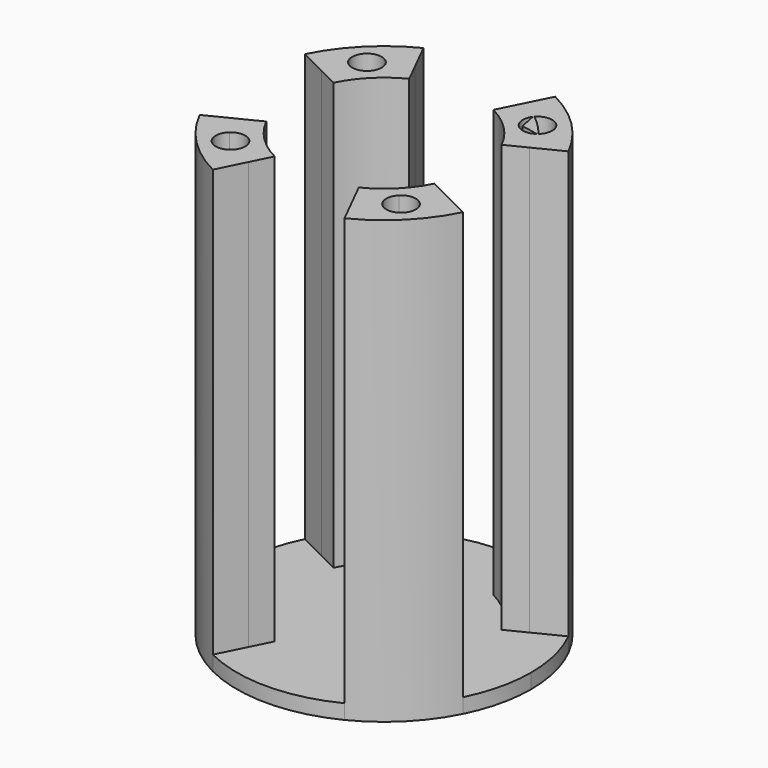
from build123d import *
from build123d import SkipClean  # not in build123d's __all__

# Parameters (mm, degrees)
F1_DEPTH = 5.08
F2_DEPTH = 152.4
F4_DEPTH = 50.8


with BuildPart() as f1:
    # F0 (on Top) → F1 (new body)
    with BuildSketch(Plane.XY):
        with BuildLine():
            Line((-29.00712, 14.50356), (0, 0))
            Line((0, 0), (-14.50356, 29.00712))
            ThreePointArc((-14.50356, 29.00712), (-22.932142, 22.932142), (-29.00712, 14.50356))
        make_face()
        with BuildLine():
            Line((-14.50356, 29.00712), (0, 0))
            Line((0, 0), (0, 32.430946))
            ThreePointArc((0, 32.430946), (-7.451105, 31.563386), (-14.50356, 29.00712))
        make_face()
        with BuildLine():
            Line((0, 32.430946), (0, 0))
            Line((0, 0), (14.50356, 29.00712))
            ThreePointArc((14.50356, 29.00712), (7.451105, 31.563386), (0, 32.430946))
        make_face()
        with BuildLine():
            Line((14.50356, 29.00712), (0, 0))
            Line((0, 0), (22.932142, 22.932142))
            ThreePointArc((22.932142, 22.932142), (18.962708, 26.309352), (14.50356, 29.00712))
        make_face()
        with BuildLine():
            Line((22.932142, 22.932142), (0, 0))
            Line((0, 0), (29.00712, 14.50356))
            ThreePointArc((29.00712, 14.50356), (26.309352, 18.962708), (22.932142, 22.932142))
        make_face()
        with BuildLine():
            Line((29.00712, 14.50356), (0, 0))
            Line((0, 0), (32.430946, 0))
            ThreePointArc((32.430946, 0), (31.563386, 7.451105), (29.00712, 14.50356))
        make_face()
        with BuildLine():
            Line((32.430946, 0), (0, 0))
            Line((0, 0), (29.00712, -14.50356))
            ThreePointArc((29.00712, -14.50356), (31.563386, -7.451105), (32.430946, 0))
        make_face()
        with BuildLine():
            Line((29.00712, -14.50356), (0, 0))
            Line((0, 0), (14.50356, -29.00712))
            ThreePointArc((14.50356, -29.00712), (22.932142, -22.932142), (29.00712, -14.50356))
        make_face()
        with BuildLine():
            Line((14.50356, -29.00712), (0, 0))
            Line((0, 0), (-14.50356, -29.00712))
            ThreePointArc((-14.50356, -29.00712), (0, -32.430946), (14.50356, -29.00712))
        make_face()
        with BuildLine():
            Line((-14.50356, -29.00712), (0, 0))
            Line((0, 0), (-29.00712, -14.50356))
            ThreePointArc((-29.00712, -14.50356), (-22.932142, -22.932142), (-14.50356, -29.00712))
        make_face()
        with BuildLine():
            Line((-29.00712, -14.50356), (0, 0))
            Line((0, 0), (-29.00712, 14.50356))
            ThreePointArc((-29.00712, 14.50356), (-32.430946, 0), (-29.00712, -14.50356))
        make_face()
        with BuildLine():
            ThreePointArc((-29.00712, -14.50356), (-32.430946, 0), (-29.00712, 14.50356))
            Line((-29.00712, 14.50356), (-35.921024, 17.960512))
            ThreePointArc((-35.921024, 17.960512), (-40.160926, 0), (-35.921024, -17.960512))
            Line((-35.921024, -17.960512), (-29.00712, -14.50356))
        make_face()
        with BuildLine():
            ThreePointArc((-29.00712, 14.50356), (-22.932142, 22.932142), (-14.50356, 29.00712))
            Line((-14.50356, 29.00712), (-17.960512, 35.921024))
            ThreePointArc((-17.960512, 35.921024), (-28.398063, 28.398063), (-35.921024, 17.960512))
            Line((-35.921024, 17.960512), (-29.00712, 14.50356))
        make_face()
        with BuildLine():
            ThreePointArc((-14.50356, 29.00712), (-7.451105, 31.563386), (0, 32.430946))
            Line((0, 32.430946), (0, 35.921024))
            Line((0, 35.921024), (17.960512, 35.921024))
            ThreePointArc((17.960512, 35.921024), (0, 40.160926), (-17.960512, 35.921024))
            Line((-17.960512, 35.921024), (-14.50356, 29.00712))
        make_face()
        with BuildLine():
            Line((0, 35.921024), (0, 32.430946))
            ThreePointArc((0, 32.430946), (7.451105, 31.563386), (14.50356, 29.00712))
            Line((14.50356, 29.00712), (17.960512, 35.921024))
            Line((17.960512, 35.921024), (0, 35.921024))
        make_face()
        with BuildLine():
            ThreePointArc((14.50356, 29.00712), (18.962708, 26.309352), (22.932142, 22.932142))
            Line((22.932142, 22.932142), (28.398063, 28.398063))
            ThreePointArc((28.398063, 28.398063), (23.482507, 32.580238), (17.960512, 35.921024))
            Line((17.960512, 35.921024), (14.50356, 29.00712))
        make_face()
        with BuildLine():
            ThreePointArc((17.960512, 35.921024), (23.482507, 32.580238), (28.398063, 28.398063))
            Line((28.398063, 28.398063), (35.921024, 35.921024))
            Line((35.921024, 35.921024), (17.960512, 35.921024))
        make_face()
        with BuildLine():
            Line((35.921024, 35.921024), (28.398063, 28.398063))
            ThreePointArc((28.398063, 28.398063), (32.580238, 23.482507), (35.921024, 17.960512))
            Line((35.921024, 17.960512), (35.921024, 35.921024))
        make_face()
        with BuildLine():
            Line((28.398063, 28.398063), (22.932142, 22.932142))
            ThreePointArc((22.932142, 22.932142), (26.309352, 18.962708), (29.00712, 14.50356))
            Line((29.00712, 14.50356), (35.921024, 17.960512))
            ThreePointArc((35.921024, 17.960512), (32.580238, 23.482507), (28.398063, 28.398063))
        make_face()
        with BuildLine():
            ThreePointArc((29.00712, 14.50356), (31.563386, 7.451105), (32.430946, 0))
            Line((32.430946, 0), (35.921024, 0))
            Line((35.921024, 0), (35.921024, 17.960512))
            Line((35.921024, 17.960512), (29.00712, 14.50356))
        make_face()
        with BuildLine():
            Line((35.921024, 0), (32.430946, 0))
            ThreePointArc((32.430946, 0), (31.563386, -7.451105), (29.00712, -14.50356))
            Line((29.00712, -14.50356), (35.921024, -17.960512))
            ThreePointArc((35.921024, -17.960512), (39.086581, -9.22709), (40.160926, 0))
            ThreePointArc((40.160926, 0), (39.086581, 9.22709), (35.921024, 17.960512))
            Line((35.921024, 17.960512), (35.921024, 0))
        make_face()
        with BuildLine():
            ThreePointArc((29.00712, -14.50356), (22.932142, -22.932142), (14.50356, -29.00712))
            Line((14.50356, -29.00712), (17.960512, -35.921024))
            ThreePointArc((17.960512, -35.921024), (28.398063, -28.398063), (35.921024, -17.960512))
            Line((35.921024, -17.960512), (29.00712, -14.50356))
        make_face()
        with BuildLine():
            ThreePointArc((14.50356, -29.00712), (0, -32.430946), (-14.50356, -29.00712))
            Line((-14.50356, -29.00712), (-17.960512, -35.921024))
            ThreePointArc((-17.960512, -35.921024), (0, -40.160926), (17.960512, -35.921024))
            Line((17.960512, -35.921024), (14.50356, -29.00712))
        make_face()
        with BuildLine():
            ThreePointArc((-14.50356, -29.00712), (-22.932142, -22.932142), (-29.00712, -14.50356))
            Line((-29.00712, -14.50356), (-35.921024, -17.960512))
            ThreePointArc((-35.921024, -17.960512), (-28.398063, -28.398063), (-17.960512, -35.921024))
            Line((-17.960512, -35.921024), (-14.50356, -29.00712))
        make_face()
        with BuildLine():
            ThreePointArc((-17.960512, -35.921024), (-28.398063, -28.398063), (-35.921024, -17.960512))
            Line((-35.921024, -17.960512), (-45.436901, -22.718451))
            ThreePointArc((-45.436901, -22.718451), (-35.921024, -35.921024), (-22.718451, -45.436901))
            Line((-22.718451, -45.436901), (-17.960512, -35.921024))
        make_face()
        with BuildLine():
            ThreePointArc((-35.921024, -17.960512), (-40.160926, 0), (-35.921024, 17.960512))
            Line((-35.921024, 17.960512), (-45.436901, 22.718451))
            ThreePointArc((-45.436901, 22.718451), (-50.8, 0), (-45.436901, -22.718451))
            Line((-45.436901, -22.718451), (-35.921024, -17.960512))
        make_face()
        with BuildLine():
            ThreePointArc((-35.921024, 17.960512), (-28.398063, 28.398063), (-17.960512, 35.921024))
            Line((-17.960512, 35.921024), (-22.718451, 45.436901))
            ThreePointArc((-22.718451, 45.436901), (-35.921024, 35.921024), (-45.436901, 22.718451))
            Line((-45.436901, 22.718451), (-35.921024, 17.960512))
        make_face()
        with BuildLine():
            ThreePointArc((-17.960512, 35.921024), (0, 40.160926), (17.960512, 35.921024))
            Line((17.960512, 35.921024), (22.718451, 45.436901))
            ThreePointArc((22.718451, 45.436901), (0, 50.8), (-22.718451, 45.436901))
            Line((-22.718451, 45.436901), (-17.960512, 35.921024))
        make_face()
        with BuildLine():
            Line((22.718451, 45.436901), (17.960512, 35.921024))
            Line((17.960512, 35.921024), (35.921024, 35.921024))
            ThreePointArc((35.921024, 35.921024), (29.703282, 41.211103), (22.718451, 45.436901))
        make_face()
        with BuildLine():
            Line((35.921024, 35.921024), (35.921024, 17.960512))
            Line((35.921024, 17.960512), (45.436901, 22.718451))
            ThreePointArc((45.436901, 22.718451), (41.211103, 29.703282), (35.921024, 35.921024))
        make_face()
        with BuildLine():
            Line((45.436901, 22.718451), (35.921024, 17.960512))
            ThreePointArc((35.921024, 17.960512), (39.086581, 9.22709), (40.160926, 0))
            ThreePointArc((40.160926, 0), (39.086581, -9.22709), (35.921024, -17.960512))
            Line((35.921024, -17.960512), (45.436901, -22.718451))
            ThreePointArc((45.436901, -22.718451), (49.441049, -11.671448), (50.8, 0))
            ThreePointArc((50.8, 0), (49.441049, 11.671448), (45.436901, 22.718451))
        make_face()
        with BuildLine():
            ThreePointArc((35.921024, -17.960512), (28.398063, -28.398063), (17.960512, -35.921024))
            Line((17.960512, -35.921024), (22.718451, -45.436901))
            ThreePointArc((22.718451, -45.436901), (35.921024, -35.921024), (45.436901, -22.718451))
            Line((45.436901, -22.718451), (35.921024, -17.960512))
        make_face()
        with BuildLine():
            ThreePointArc((17.960512, -35.921024), (0, -40.160926), (-17.960512, -35.921024))
            Line((-17.960512, -35.921024), (-22.718451, -45.436901))
            ThreePointArc((-22.718451, -45.436901), (0, -50.8), (22.718451, -45.436901))
            Line((22.718451, -45.436901), (17.960512, -35.921024))
        make_face()
    extrude(amount=F1_DEPTH)

    # F0 (on Top) → F2 (join)
    with BuildSketch(Plane.XY):
        with BuildLine():
            ThreePointArc((-14.50356, -29.00712), (-22.932142, -22.932142), (-29.00712, -14.50356))
            Line((-29.00712, -14.50356), (-35.921024, -17.960512))
            ThreePointArc((-35.921024, -17.960512), (-28.398063, -28.398063), (-17.960512, -35.921024))
            Line((-17.960512, -35.921024), (-14.50356, -29.00712))
        make_face()
        with BuildLine():
            ThreePointArc((-17.960512, -35.921024), (-28.398063, -28.398063), (-35.921024, -17.960512))
            Line((-35.921024, -17.960512), (-45.436901, -22.718451))
            ThreePointArc((-45.436901, -22.718451), (-35.921024, -35.921024), (-22.718451, -45.436901))
            Line((-22.718451, -45.436901), (-17.960512, -35.921024))
        make_face()
        with BuildLine():
            ThreePointArc((-29.00712, 14.50356), (-22.932142, 22.932142), (-14.50356, 29.00712))
            Line((-14.50356, 29.00712), (-17.960512, 35.921024))
            ThreePointArc((-17.960512, 35.921024), (-28.398063, 28.398063), (-35.921024, 17.960512))
            Line((-35.921024, 17.960512), (-29.00712, 14.50356))
        make_face()
        with BuildLine():
            ThreePointArc((-35.921024, 17.960512), (-28.398063, 28.398063), (-17.960512, 35.921024))
            Line((-17.960512, 35.921024), (-22.718451, 45.436901))
            ThreePointArc((-22.718451, 45.436901), (-35.921024, 35.921024), (-45.436901, 22.718451))
            Line((-45.436901, 22.718451), (-35.921024, 17.960512))
        make_face()
        with BuildLine():
            Line((22.718451, 45.436901), (17.960512, 35.921024))
            Line((17.960512, 35.921024), (35.921024, 35.921024))
            ThreePointArc((35.921024, 35.921024), (29.703282, 41.211103), (22.718451, 45.436901))
        make_face()
        with BuildLine():
            ThreePointArc((17.960512, 35.921024), (23.482507, 32.580238), (28.398063, 28.398063))
            Line((28.398063, 28.398063), (35.921024, 35.921024))
            Line((35.921024, 35.921024), (17.960512, 35.921024))
        make_face()
        with BuildLine():
            Line((35.921024, 35.921024), (28.398063, 28.398063))
            ThreePointArc((28.398063, 28.398063), (32.580238, 23.482507), (35.921024, 17.960512))
            Line((35.921024, 17.960512), (35.921024, 35.921024))
        make_face()
        with BuildLine():
            Line((35.921024, 35.921024), (35.921024, 17.960512))
            Line((35.921024, 17.960512), (45.436901, 22.718451))
            ThreePointArc((45.436901, 22.718451), (41.211103, 29.703282), (35.921024, 35.921024))
        make_face()
        with BuildLine():
            ThreePointArc((35.921024, -17.960512), (28.398063, -28.398063), (17.960512, -35.921024))
            Line((17.960512, -35.921024), (22.718451, -45.436901))
            ThreePointArc((22.718451, -45.436901), (35.921024, -35.921024), (45.436901, -22.718451))
            Line((45.436901, -22.718451), (35.921024, -17.960512))
        make_face()
        with BuildLine():
            ThreePointArc((14.50356, 29.00712), (18.962708, 26.309352), (22.932142, 22.932142))
            Line((22.932142, 22.932142), (28.398063, 28.398063))
            ThreePointArc((28.398063, 28.398063), (23.482507, 32.580238), (17.960512, 35.921024))
            Line((17.960512, 35.921024), (14.50356, 29.00712))
        make_face()
        with BuildLine():
            Line((28.398063, 28.398063), (22.932142, 22.932142))
            ThreePointArc((22.932142, 22.932142), (26.309352, 18.962708), (29.00712, 14.50356))
            Line((29.00712, 14.50356), (35.921024, 17.960512))
            ThreePointArc((35.921024, 17.960512), (32.580238, 23.482507), (28.398063, 28.398063))
        make_face()
        with BuildLine():
            ThreePointArc((29.00712, -14.50356), (22.932142, -22.932142), (14.50356, -29.00712))
            Line((14.50356, -29.00712), (17.960512, -35.921024))
            ThreePointArc((17.960512, -35.921024), (28.398063, -28.398063), (35.921024, -17.960512))
            Line((35.921024, -17.960512), (29.00712, -14.50356))
        make_face()
    with SkipClean():  # cleaning this boolean's faces spoils the solid; the shape is the same uncleaned
        extrude(amount=F2_DEPTH)

    # F3 (on face) → F4 (cut)
    with BuildSketch(Plane.XY.offset(152.4)):
        with BuildLine():
            ThreePointArc((-29.426583, 29.426583), (-27.57567, 31.167772), (-25.621934, 32.792745))
            ThreePointArc((-25.621934, 32.792745), (-33.018686, 33.018686), (-32.792745, 25.621934))
            ThreePointArc((-32.792745, 25.621934), (-31.167772, 27.57567), (-29.426583, 29.426583))
        make_face()
        with BuildLine():
            ThreePointArc((-29.426583, 29.426583), (-31.167772, 27.57567), (-32.792745, 25.621934))
            ThreePointArc((-32.792745, 25.621934), (-29.271482, 24.348952), (-25.834481, 25.834481))
            Line((-25.834481, 25.834481), (-29.426583, 29.426583))
        make_face()
        with BuildLine():
            ThreePointArc((-24.346583, 29.426583), (-24.676109, 31.226414), (-25.621934, 32.792745))
            ThreePointArc((-25.621934, 32.792745), (-27.57567, 31.167772), (-29.426583, 29.426583))
            Line((-29.426583, 29.426583), (-25.834481, 25.834481))
            ThreePointArc((-25.834481, 25.834481), (-24.733275, 27.482551), (-24.346583, 29.426583))
        make_face()
        with BuildLine():
            ThreePointArc((29.426583, -29.426583), (31.167772, -27.57567), (32.792745, -25.621934))
            ThreePointArc((32.792745, -25.621934), (29.271482, -24.348952), (25.834481, -25.834481))
            Line((25.834481, -25.834481), (29.426583, -29.426583))
        make_face()
        with BuildLine():
            ThreePointArc((34.506583, -29.426583), (34.058349, -27.340163), (32.792745, -25.621934))
            ThreePointArc((32.792745, -25.621934), (31.167772, -27.57567), (29.426583, -29.426583))
            Line((29.426583, -29.426583), (25.834481, -25.834481))
            ThreePointArc((25.834481, -25.834481), (27.482551, -34.119891), (34.506583, -29.426583))
        make_face()
        with BuildLine():
            ThreePointArc((-25.834481, -25.834481), (-29.271482, -24.348952), (-32.792745, -25.621934))
            ThreePointArc((-32.792745, -25.621934), (-31.167772, -27.57567), (-29.426583, -29.426583))
            Line((-29.426583, -29.426583), (-25.834481, -25.834481))
        make_face()
        with BuildLine():
            ThreePointArc((-29.426583, -29.426583), (-31.167772, -27.57567), (-32.792745, -25.621934))
            ThreePointArc((-32.792745, -25.621934), (-31.513004, -34.058349), (-24.346583, -29.426583))
            ThreePointArc((-24.346583, -29.426583), (-24.733275, -27.482551), (-25.834481, -25.834481))
            Line((-25.834481, -25.834481), (-29.426583, -29.426583))
        make_face()
        with BuildLine():
            ThreePointArc((33.018686, 33.018686), (29.271482, 34.504215), (25.621934, 32.792745))
            ThreePointArc((25.621934, 32.792745), (27.57567, 31.167772), (29.426583, 29.426583))
            Line((29.426583, 29.426583), (33.018686, 33.018686))
        make_face()
        with BuildLine():
            Line((26.556739, 26.556739), (25.355564, 32.465202))
            ThreePointArc((25.355564, 32.465202), (24.354649, 29.712744), (25.039608, 26.865169))
            Line((25.039608, 26.865169), (26.556739, 26.556739))
        make_face()
        with BuildLine():
            Line((25.834481, 25.834481), (26.556739, 26.556739))
            Line((26.556739, 26.556739), (25.039608, 26.865169))
            ThreePointArc((25.039608, 26.865169), (25.403897, 26.324262), (25.834481, 25.834481))
        make_face()
        with BuildLine():
            Line((26.865169, 25.039608), (26.556739, 26.556739))
            Line((26.556739, 26.556739), (25.834481, 25.834481))
            ThreePointArc((25.834481, 25.834481), (26.324262, 25.403897), (26.865169, 25.039608))
        make_face()
        with BuildLine():
            Line((32.465202, 25.355564), (26.556739, 26.556739))
            Line((26.556739, 26.556739), (26.865169, 25.039608))
            ThreePointArc((26.865169, 25.039608), (29.712744, 24.354649), (32.465202, 25.355564))
        make_face()
        with BuildLine():
            Line((34.506583, 29.426583), (29.426583, 29.426583))
            ThreePointArc((29.426583, 29.426583), (31.167772, 27.57567), (32.792745, 25.621934))
            ThreePointArc((32.792745, 25.621934), (34.058349, 27.340163), (34.506583, 29.426583))
        make_face()
        with BuildLine():
            ThreePointArc((34.506583, 29.426583), (34.119891, 31.370615), (33.018686, 33.018686))
            Line((33.018686, 33.018686), (29.426583, 29.426583))
            Line((29.426583, 29.426583), (34.506583, 29.426583))
        make_face()
    extrude(amount=-F4_DEPTH, mode=Mode.SUBTRACT)


solid = f1.part
